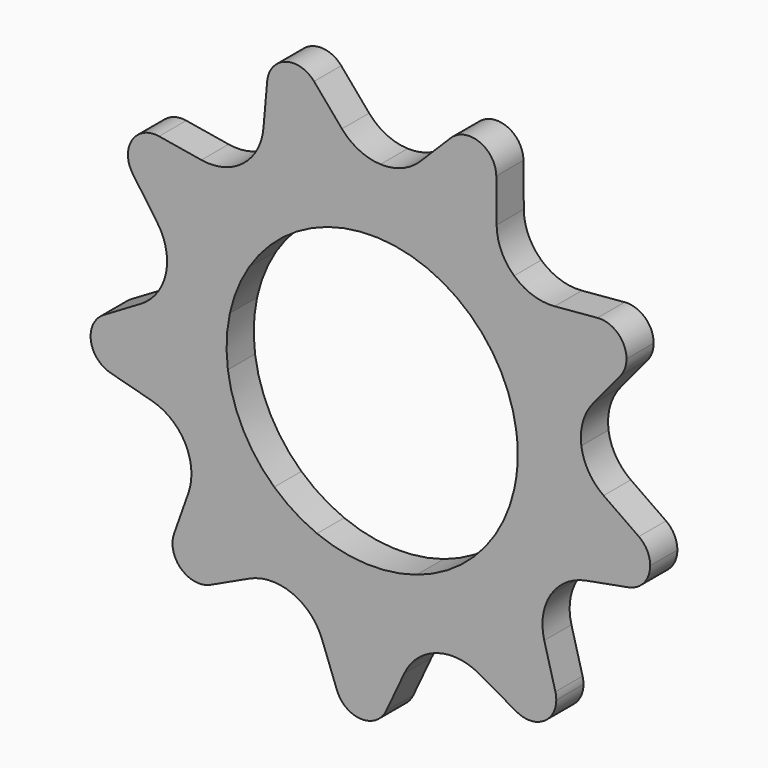
from build123d import *

# Parameters (mm, degrees)
F1_DEPTH = 14


# Not quite as in the source:
# - ends of sketch curves that miss each other by under 0.0002 mm in the source are joined


with BuildPart() as f1:
    # F0 (on Front) → F1 (new body)
    with BuildSketch(Plane.XZ):
        with BuildLine():
            ThreePointArc((32.3720842786, 105.8801466631), (29.3660148862, 95.9331361741), (35.9835922354, 87.9214484062))
            ThreePointArc((35.9835922354, 87.9214484062), (46.2807034104, 88.9685979346), (51.1501134416, 98.1018266427))
            ThreePointArc((51.1501134416, 98.1018266427), (51.1500147285, 98.1484278976), (51.1497185912, 98.1950283161))
            ThreePointArc((51.1497185912, 98.1950283161), (44.3166346477, 108.2822048792), (32.3720842786, 105.8801466631))
        make_face()
        with BuildLine():
            ThreePointArc((32.9533949945, 80.5175369614), (46.4344825558, 73.5719975927), (58.5046818367, 64.3910102669))
            ThreePointArc((58.5046818367, 64.3910102669), (53.2187863313, 71.68567665), (51.2997586494, 80.4873913517))
            Line((51.2997586494, 80.4873913517), (51.1497185912, 98.1950283161))
            ThreePointArc((51.1497185912, 98.1950283161), (51.1500147285, 98.1484278976), (51.1501134416, 98.1018266427))
            ThreePointArc((51.1501134416, 98.1018266427), (46.2807034104, 88.9685979346), (35.9835922354, 87.9214484062))
            Line((35.9835922354, 87.9214484062), (32.9533949945, 80.5175369614))
        make_face()
        with BuildLine():
            ThreePointArc((3.4274426795, 86.9324602015), (18.4710353665, 85.0165916306), (32.9533949945, 80.5175369614))
            Line((32.9533949945, 80.5175369614), (35.9835922354, 87.9214484062))
            ThreePointArc((35.9835922354, 87.9214484062), (29.3660148862, 95.9331361741), (32.3720842786, 105.8801466631))
            Line((32.3720842786, 105.8801466631), (19.8502105167, 93.3587411362))
            ThreePointArc((19.8502105167, 93.3587411362), (12.3109167385, 88.4280317588), (3.4274426795, 86.9324602015))
        make_face()
        with BuildLine():
            Line((22.7264793065, 55.5293358355), (32.9533949945, 80.5175369614))
            ThreePointArc((32.9533949945, 80.5175369614), (18.4710353665, 85.0165916306), (3.4274426795, 86.9324602015))
            Line((3.4274426795, 86.9324602015), (2.3637534996, 59.9534208315))
            ThreePointArc((2.3637534996, 59.9534208315), (12.7386450449, 58.6321321668), (22.7264793065, 55.5293358355))
        make_face()
        with BuildLine():
            Line((40.348056302, 44.407593412), (58.5046816379, 64.3910104474))
            ThreePointArc((58.5046816379, 64.3910104474), (46.4344825558, 73.5719975927), (32.9533949945, 80.5175369614))
            Line((32.9533949945, 80.5175369614), (22.7264793065, 55.5293358355))
            ThreePointArc((22.7264793065, 55.5293358355), (32.0237809946, 50.739308734), (40.348056302, 44.407593412))
        make_face()
        with BuildLine():
            ThreePointArc((58.5046818367, 64.3910102669), (68.7972457691, 53.2535348554), (76.9994402387, 40.4979777634))
            Line((76.9994402387, 40.4979777634), (84.0798485365, 44.2219297416))
            ThreePointArc((84.0798485365, 44.2219297416), (84.1603038112, 54.6129353624), (92.8569016607, 60.3005233139))
            Line((92.8569016607, 60.3005233139), (75.2159855194, 58.7574754942))
            ThreePointArc((75.2159855194, 58.7574754942), (66.2711525981, 59.8264975753), (58.5046818367, 64.3910102669))
        make_face()
        with BuildLine():
            ThreePointArc((92.8569016607, 60.3005233139), (84.1603038112, 54.6129353624), (84.0798485365, 44.2219297416))
            ThreePointArc((84.0798485365, 44.2219297416), (92.687333506, 38.4003600768), (102.3015052283, 42.3433504341))
            ThreePointArc((102.3015052283, 42.3433504341), (104.1678745826, 45.6239667523), (104.815409946, 49.3423637117))
            ThreePointArc((104.815409946, 49.3423637117), (101.2469780464, 57.4523449428), (92.8569016607, 60.3005233139))
        make_face()
        with BuildLine():
            ThreePointArc((76.9994402387, 40.4979777634), (82.8620458637, 26.5119096875), (86.2069300455, 11.7202906163))
            ThreePointArc((86.2069300455, 11.7202906163), (86.8466202271, 20.7060376023), (91.0341929436, 28.6820696464))
            Line((91.0341929436, 28.6820696464), (102.3015052283, 42.3433504341))
            ThreePointArc((102.3015052283, 42.3433504341), (92.687333506, 38.4003600768), (84.0798485365, 44.2219297416))
            Line((84.0798485365, 44.2219297416), (76.9994402387, 40.4979777634))
        make_face()
        with BuildLine():
            Line((53.1030622336, 27.9296398368), (76.9994402387, 40.4979777634))
            ThreePointArc((76.9994402387, 40.4979777634), (68.7972457691, 53.2535348554), (58.5046818367, 64.3910102669))
            Line((58.5046818367, 64.3910102669), (40.348056302, 44.407593412))
            ThreePointArc((40.348056302, 44.407593412), (47.4463763358, 36.7265758355), (53.1030622336, 27.9296398368))
        make_face()
        with BuildLine():
            Line((59.4530551421, 8.0829594997), (86.206929956, 11.7202912746))
            ThreePointArc((86.206929956, 11.7202912746), (82.8620458637, 26.5119096875), (76.9994402387, 40.4979777634))
            Line((76.9994402387, 40.4979777634), (53.1030622336, 27.9296398368))
            ThreePointArc((53.1030622336, 27.9296398368), (57.1462384569, 18.2840758647), (59.4530551421, 8.0829594997))
        make_face()
        with BuildLine():
            ThreePointArc((85.0165916418, -18.4710353151), (86.5027267571, -9.2886093459), (87, 0))
            ThreePointArc((87, 0), (86.8015060755, 5.8735460346), (86.2069300455, 11.7202906163))
            Line((86.2069300455, 11.7202906163), (59.4530551421, 8.0829594997))
            ThreePointArc((59.4530551421, 8.0829594997), (59.8631076228, 4.0507216317), (60, 0))
            ThreePointArc((60, 0), (59.657052936, -6.40593748), (58.6321321668, -12.7386450449))
            Line((58.6321321668, -12.7386450449), (85.0165916418, -18.4710353151))
        make_face()
        with BuildLine():
            ThreePointArc((86.2069300455, 11.7202906163), (86.8015060755, 5.8735460346), (87, 0))
            ThreePointArc((87, 0), (86.5027267571, -9.2886093459), (85.0165916418, -18.4710353151))
            Line((85.0165916418, -18.4710353151), (92.834209264, -20.169521321))
            ThreePointArc((92.834209264, -20.169521321), (99.5750512453, -12.2612648605), (109.8929427662, -13.4943850596))
            Line((109.8929427662, -13.4943850596), (95.3873649649, -3.3370659482))
            ThreePointArc((95.3873649649, -3.3370659482), (89.2223796623, 3.2314800802), (86.2069300455, 11.7202906163))
        make_face()
        with BuildLine():
            ThreePointArc((109.8929427662, -13.4943850596), (99.5750512453, -12.2612648605), (92.834209264, -20.169521321))
            ThreePointArc((92.834209264, -20.169521321), (95.6858924447, -30.1618871019), (105.5852806145, -33.32125171))
            ThreePointArc((105.5852806145, -33.32125171), (112.0398014596, -29.5398412019), (114.5834334946, -22.5049395793))
            ThreePointArc((114.5834334946, -22.5049395793), (113.3406001425, -17.4257960485), (109.8929427662, -13.4943850596))
        make_face()
        with BuildLine():
            Line((92.834209264, -20.169521321), (85.0165916418, -18.4710353151))
            ThreePointArc((85.0165916418, -18.4710353151), (80.5175370893, -32.953394682), (73.5719980248, -46.4344818712))
            ThreePointArc((73.5719980248, -46.4344818712), (79.8379557996, -39.9621860052), (88.1727166272, -36.5439112122))
            Line((88.1727166272, -36.5439112122), (105.5852806145, -33.32125171))
            ThreePointArc((105.5852806145, -33.32125171), (95.6858924447, -30.1618871019), (92.834209264, -20.169521321))
        make_face()
        with BuildLine():
            ThreePointArc((73.5719980248, -46.4344818712), (80.5175370893, -32.953394682), (85.0165916418, -18.4710353151))
            Line((85.0165916418, -18.4710353151), (58.6321321668, -12.7386450449))
            ThreePointArc((58.6321321668, -12.7386450449), (55.5293358355, -22.7264793065), (50.739308734, -32.0237809946))
            Line((50.739308734, -32.0237809946), (73.5719980248, -46.4344818712))
        make_face()
        with BuildLine():
            ThreePointArc((53.2535349615, -68.7972456869), (64.3910106745, -58.5046813881), (73.5719980248, -46.4344818712))
            Line((73.5719980248, -46.4344818712), (50.739308734, -32.0237809946))
            ThreePointArc((50.739308734, -32.0237809946), (44.407593412, -40.348056302), (36.7265758355, -47.4463763358))
            Line((36.7265758355, -47.4463763358), (53.2535349615, -68.7972456869))
        make_face()
        with BuildLine():
            ThreePointArc((70.9259362309, -63.8701571461), (70.4254635991, -54.875582133), (73.5719980248, -46.4344818712))
            ThreePointArc((73.5719980248, -46.4344818712), (64.3910106745, -58.5046813881), (53.2535349615, -68.7972456869))
            Line((53.2535349615, -68.7972456869), (58.1504117396, -75.1234291983))
            ThreePointArc((58.1504117396, -75.1234291983), (68.3975255483, -73.3982829864), (75.5088546274, -80.9751206903))
            Line((75.5088546274, -80.9751206903), (70.9259362309, -63.8701571461))
        make_face()
        with BuildLine():
            ThreePointArc((75.5088546274, -80.9751206903), (68.3975255483, -73.3982829864), (58.1504117396, -75.1234291983))
            ThreePointArc((58.1504117396, -75.1234291983), (53.9119588783, -84.6110520937), (59.4645297515, -93.3944698544))
            ThreePointArc((59.4645297515, -93.3944698544), (70.4239258235, -93.3248248527), (75.8836173094, -83.8219315266))
            ThreePointArc((75.8836173094, -83.8219315266), (75.7895242066, -82.3862453661), (75.5088546274, -80.9751206903))
        make_face()
        with BuildLine():
            Line((58.1504117396, -75.1234291983), (53.2535349615, -68.7972456869))
            ThreePointArc((53.2535349615, -68.7972456869), (40.4979775935, -76.9994403281), (26.5119096382, -82.8620458795))
            ThreePointArc((26.5119096382, -82.8620458795), (35.4722238433, -81.9316592406), (44.0542462703, -84.6705898743))
            Line((44.0542462703, -84.6705898743), (59.4645297515, -93.3944698544))
            ThreePointArc((59.4645297515, -93.3944698544), (53.9119588783, -84.6110520937), (58.1504117396, -75.1234291983))
        make_face()
        with BuildLine():
            ThreePointArc((26.5119096382, -82.8620458795), (40.4979775935, -76.9994403281), (53.2535349615, -68.7972456869))
            Line((53.2535349615, -68.7972456869), (36.7265758355, -47.4463763358))
            ThreePointArc((36.7265758355, -47.4463763358), (27.9296398368, -53.1030622336), (18.2840758647, -57.1462384569))
            Line((18.2840758647, -57.1462384569), (26.5119096382, -82.8620458795))
        make_face()
        with BuildLine():
            ThreePointArc((18.2840758647, -57.1462384569), (8.0829594997, -59.4530551421), (-2.3637534996, -59.9534208315))
            Line((-2.3637534996, -59.9534208315), (-3.4274425744, -86.9324602056))
            ThreePointArc((-3.4274425744, -86.9324602056), (11.7202910843, -86.2069299819), (26.5119096382, -82.8620458795))
            Line((26.5119096382, -82.8620458795), (18.2840758647, -57.1462384569))
        make_face()
        with BuildLine():
            ThreePointArc((6.8240354841, -105.9177101356), (3.7539441497, -98.2942890824), (-3.7426097076, -94.9262496498))
            ThreePointArc((-3.7426097076, -94.9262496498), (-13.087979412, -99.4697654637), (-14.4803354569, -109.7673775901))
            ThreePointArc((-14.4803354569, -109.7673775901), (-4.6093193242, -116.9091706213), (5.793334221, -110.5666974118))
            ThreePointArc((5.793334221, -110.5666974118), (6.5632693047, -108.2986462849), (6.8240354841, -105.9177101356))
        make_face()
        with BuildLine():
            ThreePointArc((13.2774736805, -94.5176919775), (18.6756903773, -87.3057505138), (26.5119096382, -82.8620458795))
            ThreePointArc((26.5119096382, -82.8620458795), (11.7202910843, -86.2069299819), (-3.4274425744, -86.9324602056))
            Line((-3.4274425744, -86.9324602056), (-3.7426097076, -94.9262496498))
            ThreePointArc((-3.7426097076, -94.9262496498), (3.7539441497, -98.2942890824), (6.8240354841, -105.9177101356))
            ThreePointArc((6.8240354841, -105.9177101356), (6.5632693047, -108.2986462849), (5.793334221, -110.5666974118))
            Line((5.793334221, -110.5666974118), (13.2774736805, -94.5176919775))
        make_face()
        with BuildLine():
            Line((-3.7426097076, -94.9262496498), (-3.4274425744, -86.9324602056))
            ThreePointArc((-3.4274425744, -86.9324602056), (-18.4710353211, -85.0165916405), (-32.9533950059, -80.5175369568))
            ThreePointArc((-32.9533950059, -80.5175369568), (-25.4913553114, -85.5643983847), (-20.6776955249, -93.1789585254))
            Line((-20.6776955249, -93.1789585254), (-14.4803354569, -109.7673775901))
            ThreePointArc((-14.4803354569, -109.7673775901), (-13.087979412, -99.4697654637), (-3.7426097076, -94.9262496498))
        make_face()
        with BuildLine():
            ThreePointArc((-32.9533950059, -80.5175369568), (-46.4344824475, -73.571997661), (-58.5046816379, -64.3910104474))
            Line((-58.5046816379, -64.3910104474), (-63.8844224782, -70.3120229024))
            ThreePointArc((-63.8844224782, -70.3120229024), (-61.2225259157, -74.0019310175), (-60.2815661336, -78.4534150279))
            ThreePointArc((-60.2815661336, -78.4534150279), (-62.0043154825, -84.3637974485), (-66.6329516532, -88.4228876024))
            Line((-66.6329516532, -88.4228876024), (-50.5836663677, -80.9393482856))
            ThreePointArc((-50.5836663677, -80.9393482856), (-41.812645664, -78.8845874059), (-32.9533950059, -80.5175369568))
        make_face()
        with BuildLine():
            ThreePointArc((-60.2815661336, -78.4534150279), (-61.2225259157, -74.0019310175), (-63.8844224782, -70.3120229024))
            ThreePointArc((-63.8844224782, -70.3120229024), (-73.9639066787, -67.7854700899), (-81.649690774, -74.7789094228))
            ThreePointArc((-81.649690774, -74.7789094228), (-78.678709789, -86.5948071535), (-66.6329516532, -88.4228876024))
            ThreePointArc((-66.6329516532, -88.4228876024), (-62.0043154825, -84.3637974485), (-60.2815661336, -78.4534150279))
        make_face()
        with BuildLine():
            Line((-63.8844224782, -70.3120229024), (-58.5046816379, -64.3910104474))
            ThreePointArc((-58.5046816379, -64.3910104474), (-68.7972458297, -53.253534777), (-76.999440456, -40.4979773503))
            ThreePointArc((-76.999440456, -40.4979773503), (-75.1121373522, -45.464601551), (-74.4705630577, -50.7388457036))
            ThreePointArc((-74.4705630577, -50.7388457036), (-74.7888024722, -54.4672847753), (-75.734313777, -58.0878569137))
            Line((-75.734313777, -58.0878569137), (-81.649690774, -74.7789094228))
            ThreePointArc((-81.649690774, -74.7789094228), (-73.9639066787, -67.7854700899), (-63.8844224782, -70.3120229024))
        make_face()
        with BuildLine():
            ThreePointArc((-76.999440456, -40.4979773503), (-82.8620458336, -26.5119097816), (-86.206929956, -11.7202912746))
            Line((-86.206929956, -11.7202912746), (-94.1340039749, -12.7980192079))
            ThreePointArc((-94.1340039749, -12.7980192079), (-94.0588276868, -13.537262817), (-94.033730751, -14.2798951161))
            ThreePointArc((-94.033730751, -14.2798951161), (-98.3374366156, -23.0068444601), (-107.880938906, -24.9050259728))
            Line((-107.880938906, -24.9050259728), (-90.7761467477, -29.4885839902))
            ThreePointArc((-90.7761467477, -29.4885839902), (-82.7363804202, -33.5524491272), (-76.999440456, -40.4979773503))
        make_face()
        with BuildLine():
            ThreePointArc((-94.033730751, -14.2798951161), (-94.0588276868, -13.537262817), (-94.1340039749, -12.7980192079))
            ThreePointArc((-94.1340039749, -12.7980192079), (-100.2312999932, -4.3835999095), (-110.6142483426, -4.8005584616))
            ThreePointArc((-110.6142483426, -4.8005584616), (-115.933457527, -15.7617710244), (-107.880938906, -24.9050259728))
            ThreePointArc((-107.880938906, -24.9050259728), (-98.3374366156, -23.0068444601), (-94.033730751, -14.2798951161))
        make_face()
        with BuildLine():
            Line((-94.1340039749, -12.7980192079), (-86.206929956, -11.7202912746))
            ThreePointArc((-86.206929956, -11.7202912746), (-86.9324602051, 3.4274425869), (-85.0165916365, 18.4710353397))
            ThreePointArc((-85.0165916365, 18.4710353397), (-88.6910103034, 10.2459824979), (-95.3540049197, 4.1831985225))
            Line((-95.3540049197, 4.1831985225), (-110.6142483426, -4.8005584616))
            ThreePointArc((-110.6142483426, -4.8005584616), (-100.2312999932, -4.3835999095), (-94.1340039749, -12.7980192079))
        make_face()
        with BuildLine():
            ThreePointArc((-98.6502358817, 50.2661740979), (-89.3763413047, 45.5784934095), (-80.3372388289, 50.7043199082))
            ThreePointArc((-80.3372388289, 50.7043199082), (-79.0724148015, 53.5195545963), (-78.6394454301, 56.5753464239))
            ThreePointArc((-78.6394454301, 56.5753464239), (-81.2429868836, 63.6816453112), (-87.8211697714, 67.424027156))
            ThreePointArc((-87.8211697714, 67.424027156), (-98.9416520314, 62.4463729395), (-98.6502358817, 50.2661740979))
        make_face()
        with BuildLine():
            ThreePointArc((-85.0165916365, 18.4710353397), (-80.5175369567, 32.9533950061), (-73.5719976643, 46.4344824422))
            Line((-73.5719976643, 46.4344824422), (-80.3372388289, 50.7043199082))
            ThreePointArc((-80.3372388289, 50.7043199082), (-89.3763413047, 45.5784934095), (-98.6502358817, 50.2661740979))
            Line((-98.6502358817, 50.2661740979), (-88.4934591999, 35.7602164834))
            ThreePointArc((-88.4934591999, 35.7602164834), (-85.533205342, 29.7572032719), (-84.515040103, 23.1418718315))
            ThreePointArc((-84.515040103, 23.1418718315), (-84.6407873584, 20.7930281014), (-85.0165916365, 18.4710353397))
        make_face()
        with BuildLine():
            Line((-80.3372388289, 50.7043199082), (-73.5719976643, 46.4344824422))
            ThreePointArc((-73.5719976643, 46.4344824422), (-64.3910104254, 58.5046816622), (-53.2535349098, 68.7972457269))
            ThreePointArc((-53.2535349098, 68.7972457269), (-61.3552649793, 64.8583604753), (-70.3564974187, 64.496888879))
            Line((-70.3564974187, 64.496888879), (-87.8211697714, 67.424027156))
            ThreePointArc((-87.8211697714, 67.424027156), (-81.2429868836, 63.6816453112), (-78.6394454301, 56.5753464239))
            ThreePointArc((-78.6394454301, 56.5753464239), (-79.0724148015, 53.5195545963), (-80.3372388289, 50.7043199082))
        make_face()
        with BuildLine():
            ThreePointArc((-53.2535349098, 68.7972457269), (-40.4979777344, 76.999440254), (-26.5119100039, 82.8620457625))
            Line((-26.5119100039, 82.8620457625), (-28.9497867858, 90.4815442234))
            ThreePointArc((-28.9497867858, 90.4815442234), (-39.1689587709, 92.3651563918), (-43.259991113, 101.917272662))
            Line((-43.259991113, 101.917272662), (-44.8036985972, 84.2764142338))
            ThreePointArc((-44.8036985972, 84.2764142338), (-47.4097338159, 75.6531070707), (-53.2535349098, 68.7972457269))
        make_face()
        with BuildLine():
            ThreePointArc((-26.5119100039, 82.8620457625), (-11.7202912224, 86.2069299631), (3.4274426795, 86.9324602015))
            ThreePointArc((3.4274426795, 86.9324602015), (-5.3107092774, 89.1227907409), (-12.4384028502, 94.6317681259))
            Line((-12.4384028502, 94.6317681259), (-23.9355898405, 108.1001611328))
            ThreePointArc((-23.9355898405, 108.1001611328), (-21.9812798602, 104.7643332773), (-21.301867361, 100.9583546072))
            ThreePointArc((-21.301867361, 100.9583546072), (-23.4172490145, 94.4727122461), (-28.9497867858, 90.4815442234))
            Line((-28.9497867858, 90.4815442234), (-26.5119100039, 82.8620457625))
        make_face()
        with BuildLine():
            ThreePointArc((-43.259991113, 101.917272662), (-39.1689587709, 92.3651563918), (-28.9497867858, 90.4815442234))
            ThreePointArc((-28.9497867858, 90.4815442234), (-23.4172490145, 94.4727122461), (-21.301867361, 100.9583546072))
            ThreePointArc((-21.301867361, 100.9583546072), (-21.9812798602, 104.7643332773), (-23.9355898405, 108.1001611328))
            ThreePointArc((-23.9355898405, 108.1001611328), (-35.6539479362, 111.4351649909), (-43.259991113, 101.917272662))
        make_face()
        with BuildLine():
            Line((-26.5119100039, 82.8620457625), (-18.2840758647, 57.1462384569))
            ThreePointArc((-18.2840758647, 57.1462384569), (-8.0829594997, 59.4530551421), (2.3637534996, 59.9534208315))
            Line((2.3637534996, 59.9534208315), (3.4274425744, 86.9324602056))
            ThreePointArc((3.4274425744, 86.9324602056), (-11.7202912224, 86.2069299631), (-26.5119100039, 82.8620457625))
        make_face()
        with BuildLine():
            ThreePointArc((-36.7265758355, 47.4463763358), (-27.9296398368, 53.1030622336), (-18.2840758647, 57.1462384569))
            Line((-18.2840758647, 57.1462384569), (-26.5119100039, 82.8620457625))
            ThreePointArc((-26.5119100039, 82.8620457625), (-40.4979777344, 76.999440254), (-53.2535349098, 68.7972457269))
            Line((-53.2535349615, 68.7972456869), (-36.7265758355, 47.4463763358))
        make_face()
        with BuildLine():
            Line((-73.5719976643, 46.4344824422), (-50.739308734, 32.0237809946))
            ThreePointArc((-50.739308734, 32.0237809946), (-44.407593412, 40.348056302), (-36.7265758355, 47.4463763358))
            Line((-36.7265758355, 47.4463763358), (-53.2535349615, 68.7972456869))
            ThreePointArc((-53.2535349098, 68.7972457269), (-64.3910104254, 58.5046816622), (-73.5719976643, 46.4344824422))
        make_face()
        with BuildLine():
            ThreePointArc((-58.6321321668, 12.7386450449), (-55.5293358355, 22.7264793065), (-50.739308734, 32.0237809946))
            Line((-50.739308734, 32.0237809946), (-73.5719976643, 46.4344824422))
            ThreePointArc((-73.5719976643, 46.4344824422), (-80.5175369567, 32.9533950061), (-85.0165916365, 18.4710353397))
            Line((-85.0165916418, 18.4710353151), (-58.6321321668, 12.7386450449))
        make_face()
        with BuildLine():
            Line((-86.206929956, -11.7202912746), (-59.4530551421, -8.0829594997))
            ThreePointArc((-59.4530551421, -8.0829594997), (-59.9534208315, 2.3637534996), (-58.6321321668, 12.7386450449))
            Line((-58.6321321668, 12.7386450449), (-85.0165916418, 18.4710353151))
            ThreePointArc((-85.0165916365, 18.4710353397), (-86.9324602051, 3.4274425869), (-86.206929956, -11.7202912746))
        make_face()
        with BuildLine():
            ThreePointArc((-53.1030622336, -27.9296398368), (-57.1462384569, -18.2840758647), (-59.4530551421, -8.0829594997))
            Line((-59.4530551421, -8.0829594997), (-86.206929956, -11.7202912746))
            ThreePointArc((-86.206929956, -11.7202912746), (-82.8620458336, -26.5119097816), (-76.999440456, -40.4979773503))
            Line((-76.999440456, -40.4979773503), (-53.1030622336, -27.9296398368))
        make_face()
        with BuildLine():
            Line((-58.5046816379, -64.3910104474), (-40.348056302, -44.407593412))
            ThreePointArc((-40.348056302, -44.407593412), (-47.4463763358, -36.7265758355), (-53.1030622336, -27.9296398368))
            Line((-53.1030622336, -27.9296398368), (-76.9994402387, -40.4979777634))
            ThreePointArc((-76.9994402387, -40.4979777634), (-68.7972458297, -53.253534777), (-58.5046816379, -64.3910104474))
        make_face()
        with BuildLine():
            ThreePointArc((-22.7264793065, -55.5293358355), (-32.0237809946, -50.739308734), (-40.348056302, -44.407593412))
            Line((-40.348056302, -44.407593412), (-58.5046816379, -64.3910104474))
            ThreePointArc((-58.5046816379, -64.3910104474), (-46.4344824475, -73.571997661), (-32.9533950059, -80.5175369568))
            Line((-32.9533949945, -80.5175369614), (-22.7264793065, -55.5293358355))
        make_face()
        with BuildLine():
            Line((-3.4274425744, -86.9324602056), (-2.3637534996, -59.9534208315))
            ThreePointArc((-2.3637534996, -59.9534208315), (-12.7386450449, -58.6321321668), (-22.7264793065, -55.5293358355))
            Line((-22.7264793065, -55.5293358355), (-32.9533949945, -80.5175369614))
            ThreePointArc((-32.9533950059, -80.5175369568), (-18.4710353211, -85.0165916405), (-3.4274425744, -86.9324602056))
        make_face()
    extrude(amount=F1_DEPTH)


solid = f1.part
